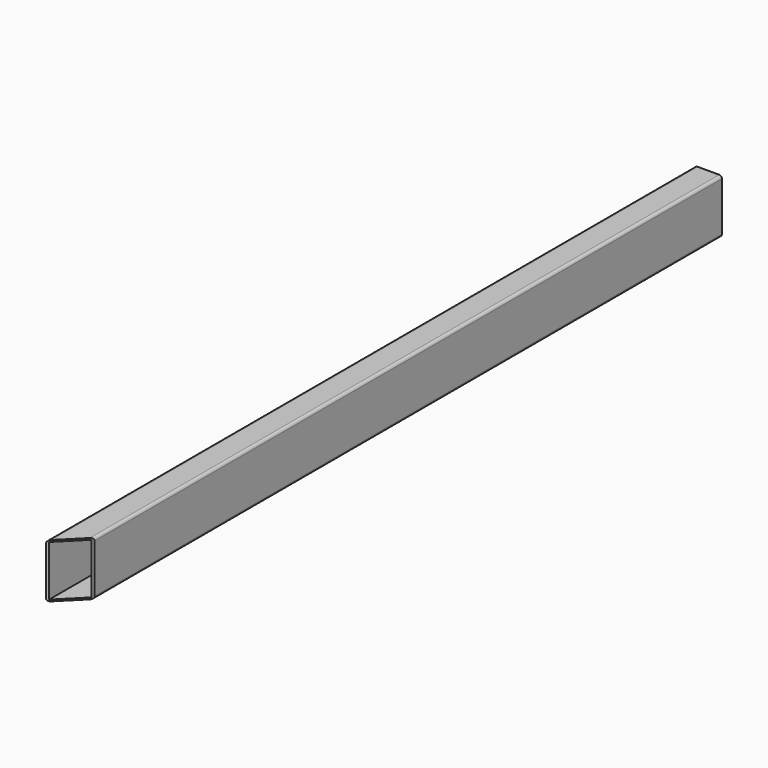
from build123d import *

# Parameters (mm, degrees)
F0_W     = 50.8
F0_H     = 101.6
F0_W_2   = 44.45
F0_H_2   = 95.25
F1_DEPTH = 1524
F3_DEPTH = 173.228
F4_R     = 5.08


# Not quite as in the source:
# - a feature names something its author has since deleted; it is built from what else it names


with BuildPart() as f1:
    # F0 (on Front) → F1 (new body)
    with BuildSketch(Plane.XZ):
        with Locations((25.4, 50.8)):
            Rectangle(F0_W, F0_H)
        with Locations((25.4, 50.8)):
            Rectangle(F0_W_2, F0_H_2, mode=Mode.SUBTRACT)
    extrude(amount=F1_DEPTH)

    # F2 (on face) → F3 (cut)
    with BuildSketch(Plane.XY.offset(101.6)):
        Polygon((50.8, -1473.2), (0, -1524), (50.8, -1524), align=None)
    extrude(amount=-F3_DEPTH, mode=Mode.SUBTRACT)

    # F4
    f4_edges = [f1.edges().sort_by_distance(p)[0] for p in [
        (0, -762, 0),
        (50.8, -736.6, 0),
        (50.8, -736.6, 101.6),
        (0, -762, 101.6),
    ]]
    fillet(f4_edges, radius=F4_R)


solid = f1.part
